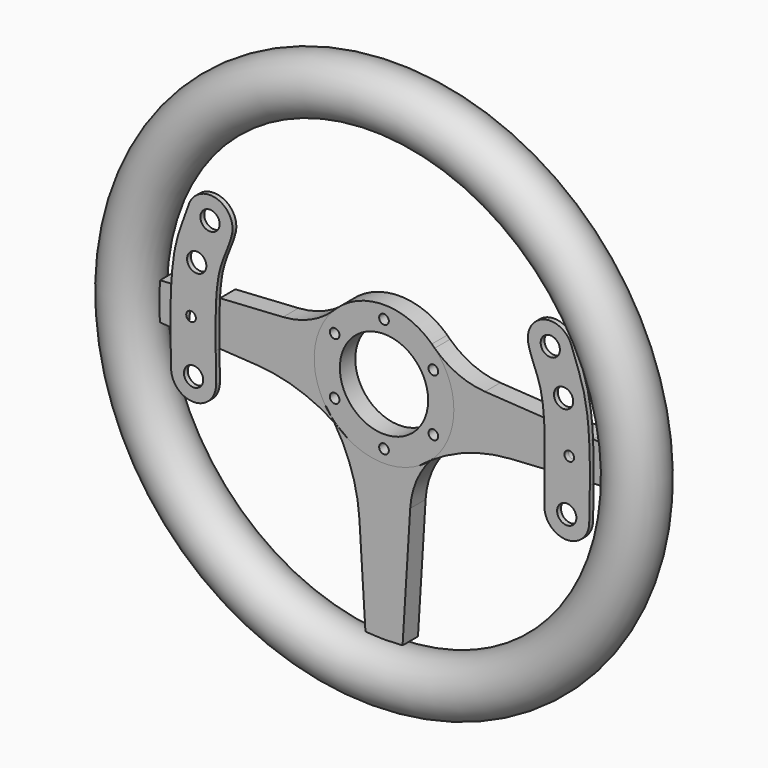
from build123d import *

# Parameters (mm, degrees)
F0_R           = 3
F0_R_2         = 6
F1_DEPTH       = 3
F2_R           = 17.5
F4_DEPTH       = 12
F0_R_3         = 27.5
F5_DEPTH       = 12
F6_D           = 6
F6_CSINK_D     = 12
F6_CSINK_ANGLE = 90


# Not quite as in the source:
# - a feature names something its author has since deleted; it is built from what else it names


with BuildPart() as f1:
    # F0 (on Front) → F1 (new body)
    with BuildSketch(Plane.XZ):
        with BuildLine():
            add(Edge.make_bspline(
                [(130.2068077697, 12.1368749286), (130.5882710118, 4.5078155701), (130.6639281343, -3.6831932109), (130.592328503, -12.1129617377)],
                knots=[0.6195482192, 0.6195482192, 0.6195482192, 0.6195482192, 0.8304216651, 0.8304216651, 0.8304216651, 0.8304216651], degree=3))
            Line((130.2068077697, 12.1368749286), (102.1695719261, 13.8759766573))
            add(Edge.make_bspline(
                [(102.1695719261, 13.8759766573), (102.6210254098, 5.5119102946), (102.5359020376, -3.9631275492), (102.4037274528, -13.861452391)],
                knots=[0.5722203527, 0.5722203527, 0.5722203527, 0.5722203527, 0.8373244665, 0.8373244665, 0.8373244665, 0.8373244665], degree=3))
            Line((102.4037274528, -13.861452391), (130.592328503, -12.1129617377))
        make_face()
        with Locations((117.7831068635, 0)):
            Circle(F0_R, mode=Mode.SUBTRACT)
        with BuildLine():
            Line((102.1695719261, 13.8759766573), (130.2068077697, 12.1368749286))
            add(Edge.make_bspline(
                [(119.3451886645, 60.5255165629), (121.4071289028, 53.8130038768), (127.6720712181, 41.1553587501), (129.7853870894, 20.5650615282), (130.2068077697, 12.1368749286)],
                knots=[0, 0, 0, 0, 0.3865862421, 0.6195482192, 0.6195482192, 0.6195482192, 0.6195482192], degree=3))
            ThreePointArc((119.3451886645, 60.5255165629), (102.3091914557, 69.9295656858), (92.3309010028, 53.2234272798))
            add(Edge.make_bspline(
                [(92.3309010028, 53.2234272798), (94.2424391466, 45.0580669711), (100.0861186212, 36.0400670766), (101.858531632, 19.6386116923), (102.1695719261, 13.8759766573)],
                knots=[0, 0, 0, 0, 0.3895701695, 0.5722203527, 0.5722203527, 0.5722203527, 0.5722203527], degree=3))
        make_face()
        with Locations((114.2406761646, 30.7705756277)):
            Circle(F0_R_2, mode=Mode.SUBTRACT)
        with Locations((105.9623516152, 56.4145954361)):
            Circle(F0_R_2, mode=Mode.SUBTRACT)
        with BuildLine():
            add(Edge.make_bspline(
                [(130.592328503, -12.1129617377), (130.5347501473, -18.8919381265), (130.3819421464, -25.825318339), (130.2163581575, -32.745027462)],
                knots=[0.8304216651, 0.8304216651, 0.8304216651, 0.8304216651, 1, 1, 1, 1], degree=3))
            Line((130.592328503, -12.1129617377), (102.4037274528, -13.861452391))
            add(Edge.make_bspline(
                [(102.4037274528, -13.861452391), (102.3226213139, -19.9353501176), (102.2237984939, -26.1686324872), (102.2203668473, -32.4024058491)],
                knots=[0.8373244665, 0.8373244665, 0.8373244665, 0.8373244665, 1, 1, 1, 1], degree=3))
            ThreePointArc((102.2203668473, -32.4024058491), (116.0490422194, -46.4090644417), (130.2163581575, -32.745027462))
        make_face()
        with Locations((116.2203647261, -32.4101127453)):
            Circle(F0_R_2, mode=Mode.SUBTRACT)
    extrude(amount=F1_DEPTH)


with BuildPart() as f1b:
    # F0 (on Front) → F1, piece 2 (new body)
    with BuildSketch(Plane.XZ):
        with BuildLine():
            add(Edge.make_bspline(
                [(-128.2011839006, 31.8213961416), (-129.224502269, 25.9292457337), (-129.8496751125, 19.279335697), (-130.2068077697, 12.1368749286)],
                knots=[0.4221247566, 0.4221247566, 0.4221247566, 0.4221247566, 0.6195482192, 0.6195482192, 0.6195482192, 0.6195482192], degree=3))
            Line((-130.2068077697, 12.1368749286), (-102.1695719261, 13.8759766573))
            add(Edge.make_bspline(
                [(-100.8108670214, 26.8158030203), (-101.4917348131, 22.9358377621), (-101.9155767017, 18.5817392437), (-102.1695719261, 13.8759766573)],
                knots=[0.4230683774, 0.4230683774, 0.4230683774, 0.4230683774, 0.5722203527, 0.5722203527, 0.5722203527, 0.5722203527], degree=3))
            add(Edge.make_bspline(
                [(-100.3122347778, 29.3568852328), (-100.4920686269, 28.5346986031), (-100.6579501674, 27.6872087292), (-100.8108670214, 26.8158030203)],
                knots=[0.3895701695, 0.3895701695, 0.3895701695, 0.3895701695, 0.4230683774, 0.4230683774, 0.4230683774, 0.4230683774], degree=3))
            add(Edge.make_bspline(
                [(-92.3309010028, 53.2234272798), (-94.2424391466, 45.0580669711), (-98.2208422082, 38.9185724034), (-100.3122347778, 29.3568852328)],
                knots=[0, 0, 0, 0, 0.3895701695, 0.3895701695, 0.3895701695, 0.3895701695], degree=3))
            ThreePointArc((-92.3309010028, 53.2234272798), (-102.3091914557, 69.9295656858), (-119.3451886645, 60.5255165629))
            add(Edge.make_bspline(
                [(-119.3451886645, 60.5255165629), (-121.4071289028, 53.8130038768), (-125.3163331133, 45.9148753492), (-127.6090926962, 34.9281517771)],
                knots=[0, 0, 0, 0, 0.3865862421, 0.3865862421, 0.3865862421, 0.3865862421], degree=3))
            add(Edge.make_bspline(
                [(-127.6090926962, 34.9281517771), (-127.819863957, 33.9181524749), (-128.0169747181, 32.8820515973), (-128.2011839006, 31.8213961416)],
                knots=[0.3865862421, 0.3865862421, 0.3865862421, 0.3865862421, 0.4221247566, 0.4221247566, 0.4221247566, 0.4221247566], degree=3))
        make_face()
        with Locations((-114.2406761646, 30.7705756277)):
            Circle(F0_R_2, mode=Mode.SUBTRACT)
        with Locations((-105.9623516152, 56.4145954361)):
            Circle(F0_R_2, mode=Mode.SUBTRACT)
        with BuildLine():
            Line((-102.1695719261, 13.8759766573), (-130.2068077697, 12.1368749286))
            add(Edge.make_bspline(
                [(-130.2068077697, 12.1368749286), (-130.5882710118, 4.5078155701), (-130.6639281343, -3.6831932109), (-130.592328503, -12.1129617377)],
                knots=[0.6195482192, 0.6195482192, 0.6195482192, 0.6195482192, 0.8304216651, 0.8304216651, 0.8304216651, 0.8304216651], degree=3))
            Line((-130.592328503, -12.1129617377), (-102.4037274528, -13.861452391))
            add(Edge.make_bspline(
                [(-102.1695719261, 13.8759766573), (-102.6210254098, 5.5119102946), (-102.5359020376, -3.9631275492), (-102.4037274528, -13.861452391)],
                knots=[0.5722203527, 0.5722203527, 0.5722203527, 0.5722203527, 0.8373244665, 0.8373244665, 0.8373244665, 0.8373244665], degree=3))
        make_face()
        with BuildLine():
            Line((-102.4037274528, -13.861452391), (-130.592328503, -12.1129617377))
            add(Edge.make_bspline(
                [(-130.592328503, -12.1129617377), (-130.5347501473, -18.8919381265), (-130.3819421464, -25.825318339), (-130.2163581575, -32.745027462)],
                knots=[0.8304216651, 0.8304216651, 0.8304216651, 0.8304216651, 1, 1, 1, 1], degree=3))
            ThreePointArc((-130.2163581575, -32.745027462), (-116.0490422194, -46.4090644417), (-102.2203668473, -32.4024058491))
            add(Edge.make_bspline(
                [(-102.4037274528, -13.861452391), (-102.3226213139, -19.9353501176), (-102.2237984939, -26.1686324872), (-102.2203668473, -32.4024058491)],
                knots=[0.8373244665, 0.8373244665, 0.8373244665, 0.8373244665, 1, 1, 1, 1], degree=3))
        make_face()
        with Locations((-116.2203647261, -32.4101127453)):
            Circle(F0_R_2, mode=Mode.SUBTRACT)
    extrude(amount=F1_DEPTH)

    # F6 (through all)
    with Locations(Plane(origin=(0, 0, 0), x_dir=(1, 0, 0), z_dir=(0, 1, 0))):
        with Locations((-117.7831068635, 0)):
            CounterSinkHole(F6_D / 2, F6_CSINK_D / 2, counter_sink_angle=F6_CSINK_ANGLE)


with BuildPart() as f3:
    # F2 (on Right) → F3 (revolve)
    with BuildSketch(Plane.YZ):
        with Locations((0, -157.5)):
            Circle(F2_R)
    revolve(axis=Axis((0, 0, 0), (0, -1, 0)))


with BuildPart() as f4:
    # F0 (on Front) → F4 (new body)
    with BuildSketch(Plane.XZ):
        with BuildLine():
            ThreePointArc((139.5219979401, -11.5590696335), (139.8804484401, -5.7844744092), (140, 0))
            ThreePointArc((140, 0), (139.8804484401, 5.7844744092), (139.5219979401, 11.5590696335))
            Line((139.5219979401, 11.5590696335), (130.2068077697, 12.1368749286))
            add(Edge.make_bspline(
                [(130.2068077697, 12.1368749286), (130.5882710118, 4.5078155701), (130.6639281343, -3.6831932109), (130.592328503, -12.1129617377)],
                knots=[0.6195482192, 0.6195482192, 0.6195482192, 0.6195482192, 0.8304216651, 0.8304216651, 0.8304216651, 0.8304216651], degree=3))
            Line((130.592328503, -12.1129617377), (139.5219979401, -11.5590696335))
        make_face()
        with BuildLine():
            add(Edge.make_bspline(
                [(130.2068077697, 12.1368749286), (130.5882710118, 4.5078155701), (130.6639281343, -3.6831932109), (130.592328503, -12.1129617377)],
                knots=[0.6195482192, 0.6195482192, 0.6195482192, 0.6195482192, 0.8304216651, 0.8304216651, 0.8304216651, 0.8304216651], degree=3))
            Line((130.2068077697, 12.1368749286), (102.1695719261, 13.8759766573))
            add(Edge.make_bspline(
                [(102.1695719261, 13.8759766573), (102.6210254098, 5.5119102946), (102.5359020376, -3.9631275492), (102.4037274528, -13.861452391)],
                knots=[0.5722203527, 0.5722203527, 0.5722203527, 0.5722203527, 0.8373244665, 0.8373244665, 0.8373244665, 0.8373244665], degree=3))
            Line((102.4037274528, -13.861452391), (130.592328503, -12.1129617377))
        make_face()
        with Locations((117.7831068635, 0)):
            Circle(F0_R, mode=Mode.SUBTRACT)
        with BuildLine():
            add(Edge.make_bspline(
                [(102.1695719261, 13.8759766573), (102.6210254098, 5.5119102946), (102.5359020376, -3.9631275492), (102.4037274528, -13.861452391)],
                knots=[0.5722203527, 0.5722203527, 0.5722203527, 0.5722203527, 0.8373244665, 0.8373244665, 0.8373244665, 0.8373244665], degree=3))
            Line((102.1695719261, 13.8759766573), (62.8689838662, 16.3137248368))
            ThreePointArc((62.8689838662, 16.3137248368), (46.0178534963, 20.3687862662), (31.5635389036, 29.9331423656))
            ThreePointArc((31.5635389036, 29.9331423656), (40.4058408049, 16.1126667205), (43.5, 0))
            ThreePointArc((43.5, 0), (40.4366510118, -16.0351880235), (31.6780572438, -29.8119219317))
            ThreePointArc((31.6780572438, -29.8119219317), (30.8180469828, -30.7001299699), (29.9331423656, -31.5635389036))
            ThreePointArc((29.9331423656, -31.5635389036), (29.6601999589, -31.8537341609), (29.3895783881, -32.1460949144))
            ThreePointArc((29.3895783881, -32.1460949144), (53.0790723601, -20.4210358444), (79.0130333362, -15.3123370931))
            Line((79.0130333362, -15.3123370931), (102.4037274528, -13.861452391))
        make_face()
    extrude(amount=-F4_DEPTH)


with BuildPart() as f4b:
    # F0 (on Front) → F4, piece 2 (new body)
    with BuildSketch(Plane.XZ):
        with BuildLine():
            Line((-130.2068077697, 12.1368749286), (-139.5219979401, 11.5590696335))
            ThreePointArc((-139.5219979401, 11.5590696335), (-140, 0), (-139.5219979401, -11.5590696335))
            Line((-139.5219979401, -11.5590696335), (-130.592328503, -12.1129617377))
            add(Edge.make_bspline(
                [(-130.2068077697, 12.1368749286), (-130.5882710118, 4.5078155701), (-130.6639281343, -3.6831932109), (-130.592328503, -12.1129617377)],
                knots=[0.6195482192, 0.6195482192, 0.6195482192, 0.6195482192, 0.8304216651, 0.8304216651, 0.8304216651, 0.8304216651], degree=3))
        make_face()
    extrude(amount=-F4_DEPTH)


with BuildPart() as f4c:
    # F0 (on Front) → F4, piece 3 (new body)
    with BuildSketch(Plane.XZ):
        with BuildLine():
            ThreePointArc((-11.5590696335, -139.5219979401), (0, -140), (11.5590696335, -139.5219979401))
            Line((11.5590696335, -139.5219979401), (16.3137248368, -62.8689838662))
            ThreePointArc((16.3137248368, -62.8689838662), (20.2113142672, -46.3837953144), (29.3895783881, -32.1460949144))
            ThreePointArc((29.3895783881, -32.1460949144), (29.2257610077, -32.2565251152), (29.0621621156, -32.3672787421))
            ThreePointArc((29.0621621156, -32.3672787421), (25.87857181, -34.9649756338), (22.464084382, -37.2507035219))
            ThreePointArc((22.464084382, -37.2507035219), (0, -43.5), (-22.464084382, -37.2507035219))
            ThreePointArc((-22.464084382, -37.2507035219), (-25.87857181, -34.9649756338), (-29.0621621156, -32.3672787421))
            ThreePointArc((-29.0621621156, -32.3672787421), (-30.0530691539, -31.7036172691), (-31.0518205428, -31.0518205428))
            ThreePointArc((-31.0518205428, -31.0518205428), (-20.1060659376, -54.0229684417), (-15.3123370931, -79.0130333362))
            Line((-15.3123370931, -79.0130333362), (-11.5590696335, -139.5219979401))
        make_face()
    extrude(amount=-F4_DEPTH)


with BuildPart() as f4d:
    # F0 (on Front) → F4, piece 4 (new body)
    with BuildSketch(Plane.XZ):
        with BuildLine():
            Line((-62.8689838662, 16.3137248368), (-102.1695719261, 13.8759766573))
            add(Edge.make_bspline(
                [(-102.1695719261, 13.8759766573), (-102.6210254098, 5.5119102946), (-102.5359020376, -3.9631275492), (-102.4037274528, -13.861452391)],
                knots=[0.5722203527, 0.5722203527, 0.5722203527, 0.5722203527, 0.8373244665, 0.8373244665, 0.8373244665, 0.8373244665], degree=3))
            Line((-102.4037274528, -13.861452391), (-79.0130333362, -15.3123370931))
            ThreePointArc((-79.0130333362, -15.3123370931), (-54.0229684417, -20.1060659376), (-31.0518205428, -31.0518205428))
            ThreePointArc((-31.0518205428, -31.0518205428), (-31.7036172691, -30.0530691539), (-32.3672787421, -29.0621621156))
            ThreePointArc((-32.3672787421, -29.0621621156), (-34.9649756338, -25.87857181), (-37.2507035219, -22.464084382))
            ThreePointArc((-37.2507035219, -22.464084382), (-43.2460094443, 4.6938967969), (-31.5635389036, 29.9331423656))
            ThreePointArc((-31.5635389036, 29.9331423656), (-46.0178534963, 20.3687862662), (-62.8689838662, 16.3137248368))
        make_face()
    extrude(amount=-F4_DEPTH)


with BuildPart() as f5:
    # F0 (on Front) → F5 (new body)
    with BuildSketch(Plane.XZ):
        with BuildLine():
            ThreePointArc((43.5, 0), (40.4058408049, 16.1126667205), (31.5635389036, 29.9331423656))
            ThreePointArc((31.5635389036, 29.9331423656), (30.6769433369, 30.7947712916), (29.8119219317, 31.6780572438))
            ThreePointArc((29.8119219317, 31.6780572438), (0, 43.5), (-29.8119219317, 31.6780572438))
            ThreePointArc((-29.8119219317, 31.6780572438), (-30.6769433369, 30.7947712916), (-31.5635389036, 29.9331423656))
            ThreePointArc((-31.5635389036, 29.9331423656), (-43.2460094443, 4.6938967969), (-37.2507035219, -22.464084382))
            ThreePointArc((-37.2507035219, -22.464084382), (-34.7412606899, -25.7129940244), (-32.3672787421, -29.0621621156))
            ThreePointArc((-32.3672787421, -29.0621621156), (-30.7591449816, -30.7591449816), (-29.0621621156, -32.3672787421))
            ThreePointArc((-29.0621621156, -32.3672787421), (-25.7129940244, -34.7412606899), (-22.464084382, -37.2507035219))
            ThreePointArc((-22.464084382, -37.2507035219), (0, -43.5), (22.464084382, -37.2507035219))
            ThreePointArc((22.464084382, -37.2507035219), (25.7129940244, -34.7412606899), (29.0621621156, -32.3672787421))
            ThreePointArc((29.0621621156, -32.3672787421), (29.50038961, -31.9683751989), (29.9331423656, -31.5635389036))
            ThreePointArc((29.9331423656, -31.5635389036), (30.7947712916, -30.6769433369), (31.6780572438, -29.8119219317))
            ThreePointArc((31.6780572438, -29.8119219317), (40.4366510118, -16.0351880235), (43.5, 0))
        make_face()
        with Locations((-30.7439018343, -17.75)):
            Circle(F0_R, mode=Mode.SUBTRACT)
        with Locations((0, -35.5)):
            Circle(F0_R, mode=Mode.SUBTRACT)
        with Locations((30.7439018343, -17.75)):
            Circle(F0_R, mode=Mode.SUBTRACT)
        with Locations((-30.7439018343, 17.75)):
            Circle(F0_R, mode=Mode.SUBTRACT)
        Circle(F0_R_3, mode=Mode.SUBTRACT)
        with Locations((30.7439018343, 17.75)):
            Circle(F0_R, mode=Mode.SUBTRACT)
        with Locations((0, 35.5)):
            Circle(F0_R, mode=Mode.SUBTRACT)
    extrude(amount=-F5_DEPTH)


solid = Compound([f1.part, f1b.part, f3.part, f4.part, f4b.part, f4c.part, f4d.part, f5.part])
